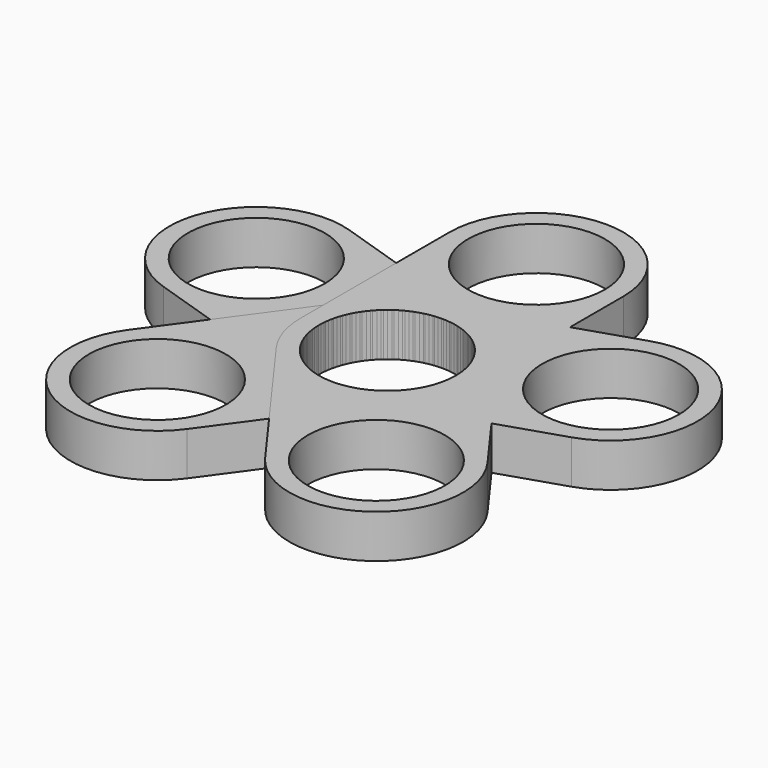
from build123d import *

# Parameters (mm, degrees)
F1_DEPTH         = 7
F1_COPIES_COUNT  = 3
F1_COPIES_ANGLE  = 144
F1_COPIES1_COUNT = 3
F1_COPIES1_ANGLE = 144


# Not quite as in the source:
# - a feature of the source that left no trace in its solid (it failed there, or was rolled back) is left out
# - a pattern or mirror of a feature is missing from the dataset's text; its kind, count and spacing are read off the source's solid


with BuildPart() as f1:
    # F0 (on Top) → F1 (new body)
    with BuildSketch(Plane.XY):
        with BuildLine():
            ThreePointArc((-2.0728331149, 7.3347839198), (8.9521668851, 18.3597839198), (19.9771668851, 7.3347839198))
            Line((19.9771668851, 7.3347839198), (22.9521668851, 7.3347839198))
            ThreePointArc((22.9521668851, 7.3347839198), (8.9521668851, 21.3347839198), (-5.0478331149, 7.3347839198))
            Line((-5.0478331149, 7.3347839198), (-2.0728331149, 7.3347839198))
        make_face()
        with BuildLine():
            Line((22.9521668851, 7.3347839198), (19.9771668851, 7.3347839198))
            ThreePointArc((19.9771668851, 7.3347839198), (8.9521668851, -3.6902160802), (-2.0728331149, 7.3347839198))
            Line((-2.0728331149, 7.3347839198), (-5.0478331149, 7.3347839198))
            ThreePointArc((-5.0478331149, 7.3347839198), (8.9521668851, -6.6652160802), (22.9521668851, 7.3347839198))
        make_face()
        with BuildLine():
            Line((22.9521668851, -22.6652160802), (22.9521668851, 7.3347839198))
            ThreePointArc((22.9521668851, 7.3347839198), (8.9521668851, -6.6652160802), (-5.0478331149, 7.3347839198))
            Line((-5.0478331149, 7.3347839198), (-5.0478331149, -22.6652160802))
            ThreePointArc((-5.0478331149, -22.6652160802), (8.9521668851, -8.6652160802), (22.9521668851, -22.6652160802))
        make_face()
        with BuildLine():
            ThreePointArc((-5.0478331149, -22.6652160802), (8.9521668851, -36.6652160802), (22.9521668851, -22.6652160802))
            Line((22.9521668851, -22.6652160802), (19.9771668851, -22.6652160802))
            ThreePointArc((19.9771668851, -22.6652160802), (8.9521668851, -33.6902160802), (-2.0728331149, -22.6652160802))
            Line((-2.0728331149, -22.6652160802), (-5.0478331149, -22.6652160802))
        make_face()
        with BuildLine():
            Line((19.9771668851, -22.6652160802), (22.9521668851, -22.6652160802))
            ThreePointArc((22.9521668851, -22.6652160802), (8.9521668851, -8.6652160802), (-5.0478331149, -22.6652160802))
            Line((-5.0478331149, -22.6652160802), (-2.0728331149, -22.6652160802))
            ThreePointArc((-2.0728331149, -22.6652160802), (8.9521668851, -11.6402160802), (19.9771668851, -22.6652160802))
        make_face()
    extrude(amount=F1_DEPTH)


with BuildPart() as f1_copies_1:
    # F1_copies: instance of F1
    add(f1.part.rotate(Axis((8.952167, -22.665216, 0), (0, 0, 1)), 1 * F1_COPIES_ANGLE / (F1_COPIES_COUNT - 1)))


with BuildPart() as f1_copies_2:
    # F1_copies: instance of F1
    add(f1.part.rotate(Axis((8.952167, -22.665216, 0), (0, 0, 1)), 2 * F1_COPIES_ANGLE / (F1_COPIES_COUNT - 1)))


with BuildPart() as f1_1:
    add(f1.part)

    # F1_copies1: F1 ×3 about axis
    f1_copies1_axis = Axis((8.952167, -22.665216, 0), (0, 0, -1))
    for i in range(1, F1_COPIES1_COUNT):
        add(f1.part.rotate(f1_copies1_axis, i * F1_COPIES1_ANGLE / (F1_COPIES1_COUNT - 1)))

    # F3: union 


solid = Compound([f1_copies_1.part, f1_copies_2.part, f1_1.part])
